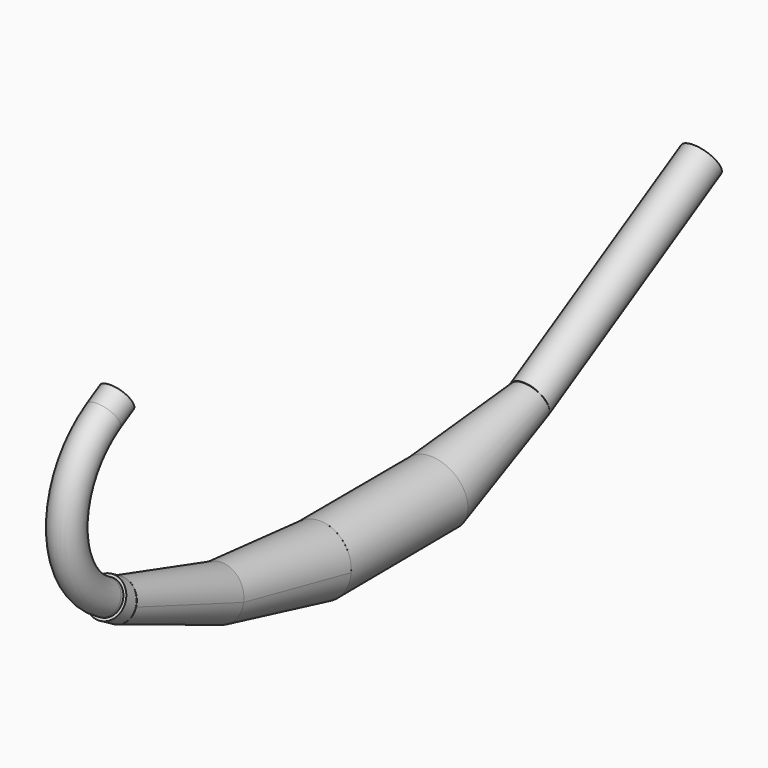
from build123d import *

# Parameters (mm, degrees)
F1_ANGLE_START = 30
F1_ANGLE       = 120
F2_DEPTH       = 25.4
F3_DEPTH       = 25.4
F6_R           = 25.0141169265
F7_DEPTH       = 25.4
F9_R           = 25.4
F11_R          = 33.61271962
F14_R          = 44.2808543302
F17_R          = 44.0697240881
F20_R          = 25.1826994789
F23_R          = 25.4
F24_REACH      = 1121.8902596119


with BuildPart() as f1:
    # F0 (on Front) → F1 (revolve)
    with BuildSketch(Plane.XZ, mode=Mode.PRIVATE) as f1_sk:
        with BuildLine():
            ThreePointArc((0, -21.43125), (15.1541822043, -15.1541822043), (21.43125, 0))
            ThreePointArc((21.43125, 0), (-15.1541822043, 15.1541822043), (0, -21.43125))
        make_face()
    revolve(f1_sk.sketch.rotate(Axis((0, 0, -121.285), (1, 0, 0)), F1_ANGLE_START), axis=Axis((0, 0, -121.285), (1, 0, 0)), revolution_arc=F1_ANGLE)

    # F2 (add): a face of the model
    f2_faces = [f1.faces().sort_by_distance(p)[0] for p in [
        (0, -60.6425, -16.249108902),
    ]]
    extrude(f2_faces, amount=F2_DEPTH)

    # F3 (add): a face of the model
    f3_faces = [f1.faces().sort_by_distance(p)[0] for p in [
        (0, -60.6425, -226.320891098),
    ]]
    extrude(f3_faces, amount=F3_DEPTH)


with BuildPart() as f7:
    # F6 (on line) → F7 (new body)
    with BuildSketch(Plane(origin=(0, 78.3347376279, -45.2265818564), x_dir=(-1, 0, 0), z_dir=(0, 0.8660254038, -0.5))):
        with Locations((0, -226.320891098)):
            Circle(F6_R)
    extrude(amount=-F7_DEPTH)

    # F9 (on line) → F12 section 0
    with BuildSketch(Plane(origin=(0, 42.6950383259, -15.5397231015), x_dir=(-1, 0, 0), z_dir=(0, 0.9396926208, -0.3420201433))):
        with Locations((0, -237.8236915488)):
            Circle(F9_R)
    # F11 (on line) → F12 section 1
    with BuildSketch(Plane(origin=(0, 175.5117654441, -30.9474596796), x_dir=(1, 0, 0), z_dir=(0, -0.984807753, 0.1736481777))):
        with Locations((0, -271.8723195376)):
            Circle(F11_R)
    loft()


with BuildPart() as f15:
    # F12_face (on face) → F15 section 0
    with BuildSketch(Plane(origin=(0, 128.3016325983, -298.6894277896), x_dir=(-1, 0, 0), z_dir=(0, 0.984807753, -0.1736481777))):
        with BuildLine():
            ThreePointArc((33.61271962, 0), (0, 33.61271962), (-33.61271962, 0))
            ThreePointArc((-33.61271962, 0), (0, -33.61271962), (33.61271962, 0))
        make_face()
    # F14 (on line) → F15 section 1
    with BuildSketch(Plane(origin=(0, 318.2347595961, -27.8419338046), x_dir=(-1, 0, 0), z_dir=(0, 0.9961946981, -0.0871557427))):
        with Locations((0, -300.5201756507)):
            Circle(F14_R)
    loft()


with BuildPart() as f18:
    # F15_face (on face) → F18 section 0
    with BuildSketch(Plane(origin=(0, 292.0427004766, -327.2185394574), x_dir=(-1, 0, 0), z_dir=(0, 0.9961946981, -0.0871557427))):
        with BuildLine():
            ThreePointArc((-44.2808543302, 0), (0, -44.2808543302), (44.2808543302, 0))
            ThreePointArc((44.2808543302, 0), (0, 44.2808543302), (-44.2808543302, 0))
        make_face()
    # F17 (on line) → F18 section 1
    with BuildSketch(Plane(origin=(0, 433.9787527242, 57.134386696), x_dir=(-1, 0, 0), z_dir=(0, 0.9914448614, 0.1305261922))):
        with Locations((0, -386.5650979544)):
            Circle(F17_R)
    loft()


with BuildPart() as f21:
    # F18_face (on face) → F21 section 0
    with BuildSketch(Plane(origin=(0, 484.4356230054, -326.1235932574), x_dir=(-1, 0, 0), z_dir=(0, 0.9914448614, 0.1305261922))):
        with BuildLine():
            ThreePointArc((-44.0697240881, 0), (0, -44.0697240881), (44.0697240881, 0))
            ThreePointArc((44.0697240881, 0), (0, 44.0697240881), (-44.0697240881, 0))
        make_face()
    # F20 (on line) → F21 section 1
    with BuildSketch(Plane(origin=(0, 447.302537817, 185.2787776477), x_dir=(-1, 0, 0), z_dir=(0, 0.9238795325, 0.3826834324))):
        with Locations((0, -506.7326347527)):
            Circle(F20_R)
    loft()


with BuildPart() as f24:
    f24_end = Plane(origin=(0, 641.2207217755, -282.8811320558), x_dir=(0, -0.3826834324, 0.9238795325), z_dir=(0, 0.9238795325, 0.3826834324))
    # F23 (on line) → F24 (new body, up to a plane its end follows)
    with BuildSketch(Plane(origin=(0, 641.5393792313, 370.3929332949), x_dir=(-1, 0, 0), z_dir=(0, 0.8660254038, 0.5))):
        with Locations((0, -565.1598654933)):
            Circle(F23_R)
    f24_long = extrude(amount=-F24_REACH, mode=Mode.PRIVATE)
    add(split(f24_long, bisect_by=f24_end, keep=Keep.TOP, mode=Mode.PRIVATE))


solid = Compound([f1.part, f7.part, f15.part, f18.part, f21.part, f24.part])
